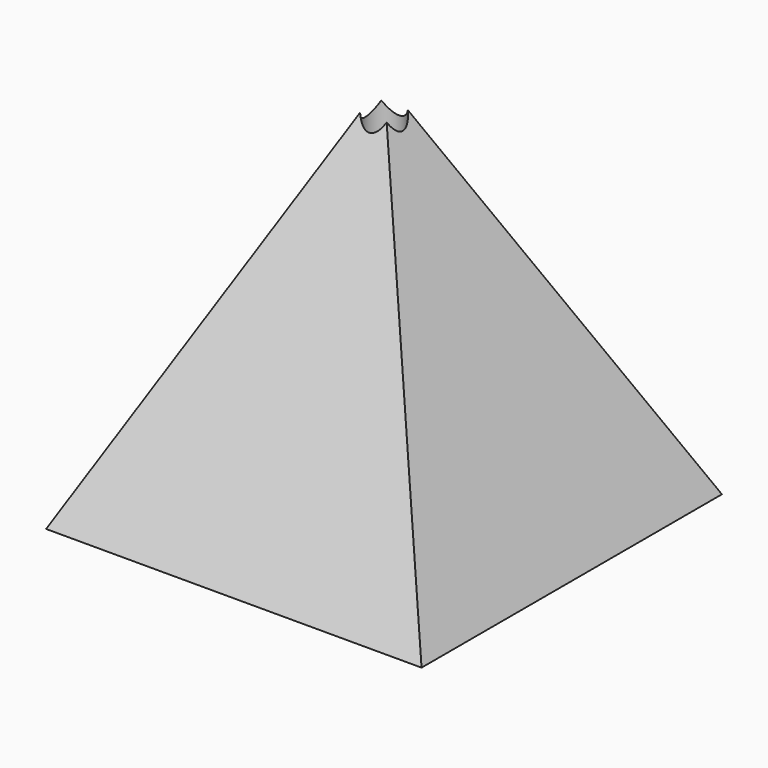
from build123d import *

# Parameters (mm, degrees)
F0_W  = 76.2
F0_H  = 76.2
F2_W  = 38.1
F2_H  = 38.1
F4_W  = 38.1
F4_H  = 38.1
F8_D  = 3.81
F10_D = 3.81


with BuildPart() as f3:
    # F0 (on Top) → F3 section 0
    with BuildSketch(Plane.XY):
        Rectangle(F0_W, F0_H)
    # F2 (on offset) → F3 section 1
    with BuildSketch(Plane.XY.offset(38.1)):
        Rectangle(F2_W, F2_H)
    loft()

    # F10 (through all)
    with Locations(Plane.XY.offset(38.1)):
        with Locations((0, 0)):
            Hole(F10_D / 2)


with BuildPart() as f6:
    # F4 (on offset) → F6 section 0
    with BuildSketch(Plane.XY.offset(38.1), mode=Mode.PRIVATE) as f6_s0:
        Rectangle(F4_W, F4_H)
    loft([f6_s0.sketch, Vertex(0, 0, 76.5771791339)])

    # F8 (through all)
    with Locations(Plane(origin=(0, 0, 38.1), x_dir=(1, 0, 0), z_dir=(0, 0, -1))):
        with Locations((0, 0)):
            Hole(F8_D / 2)


solid = f6.part
